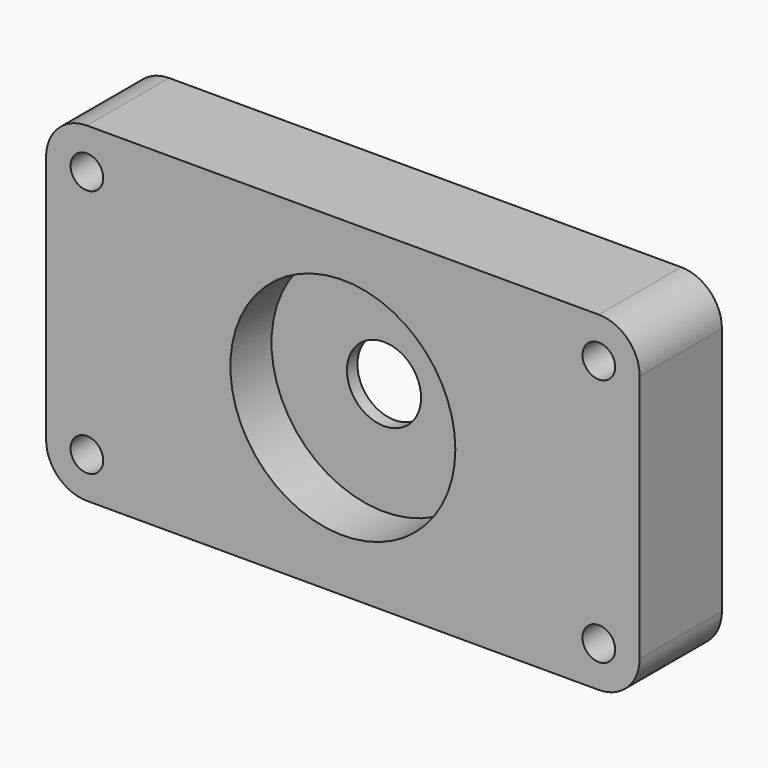
from build123d import *

# Parameters (mm, degrees)
F0_R     = 17.4971354571
F0_R_2   = 11.8450866669
F0_R_3   = 5.7656301988
F1_DEPTH = 2.032
F0_R_4   = 2.5396522034
F2_DEPTH = 8
F3_DEPTH = 8


# Not quite as in the source:
# - a feature names something its author has since deleted; it is built from what else it names


with BuildPart() as f1:
    # F0 (on Front) → F1 (new body)
    with BuildSketch(Plane.XZ):
        with Locations((3.1854841864, -0.0279111721)):
            Circle(F0_R)
        with Locations((3.1854841864, -0.0279111721)):
            Circle(F0_R_2, mode=Mode.SUBTRACT)
        with Locations((3.1854841864, -0.0279111721)):
            Circle(F0_R_2)
        with Locations((3.1854841864, -0.0279111721)):
            Circle(F0_R_3, mode=Mode.SUBTRACT)
    extrude(amount=-F1_DEPTH)

    # F0 (on Front) → F2 (join)
    with BuildSketch(Plane.XZ):
        with BuildLine():
            ThreePointArc((-42.9830769071, -19.3787951119), (-41.1232049677, -23.8689231724), (-36.6330769071, -25.7287951119))
            Line((-36.6330769071, -25.7287951119), (43.0040508678, -25.7287951119))
            ThreePointArc((43.0040508678, -25.7287951119), (47.4941789284, -23.8689231724), (49.3540508678, -19.3787951119))
            Line((49.3540508678, -19.3787951119), (49.3540508678, 19.3229727678))
            ThreePointArc((49.3540508678, 19.3229727678), (47.4941772917, 23.8131047796), (43.0040452799, 25.6729783557))
            Line((43.0040452799, 25.6729783557), (-36.6330769071, 25.6729783557))
            ThreePointArc((-36.6330769071, 25.6729783557), (-41.1232049677, 23.8131064163), (-42.9830769071, 19.3229783557))
            Line((-42.9830769071, 19.3229783557), (-42.9830769071, -19.3787951119))
        make_face()
        with Locations((-36.6330769071, -19.3787951119)):
            Circle(F0_R_4, mode=Mode.SUBTRACT)
        with Locations((3.1854841864, -0.0279111721)):
            Circle(F0_R, mode=Mode.SUBTRACT)
        with Locations((43.0040452799, -19.3787951119)):
            Circle(F0_R_4, mode=Mode.SUBTRACT)
        with Locations((-36.6330769071, 19.3229727678)):
            Circle(F0_R_4, mode=Mode.SUBTRACT)
        with Locations((43.0040452799, 19.3229727678)):
            Circle(F0_R_4, mode=Mode.SUBTRACT)
    extrude(amount=-F2_DEPTH)

    # F0 (on Front) → F3 (join)
    with BuildSketch(Plane.XZ):
        with BuildLine():
            ThreePointArc((-42.9830769071, -19.3787951119), (-41.1232049677, -23.8689231724), (-36.6330769071, -25.7287951119))
            Line((-36.6330769071, -25.7287951119), (43.0040508678, -25.7287951119))
            ThreePointArc((43.0040508678, -25.7287951119), (47.4941789284, -23.8689231724), (49.3540508678, -19.3787951119))
            Line((49.3540508678, -19.3787951119), (49.3540508678, 19.3229727678))
            ThreePointArc((49.3540508678, 19.3229727678), (47.4941772917, 23.8131047796), (43.0040452799, 25.6729783557))
            Line((43.0040452799, 25.6729783557), (-36.6330769071, 25.6729783557))
            ThreePointArc((-36.6330769071, 25.6729783557), (-41.1232049677, 23.8131064163), (-42.9830769071, 19.3229783557))
            Line((-42.9830769071, 19.3229783557), (-42.9830769071, -19.3787951119))
        make_face()
        with Locations((-36.6330769071, -19.3787951119)):
            Circle(F0_R_4, mode=Mode.SUBTRACT)
        with Locations((3.1854841864, -0.0279111721)):
            Circle(F0_R, mode=Mode.SUBTRACT)
        with Locations((43.0040452799, -19.3787951119)):
            Circle(F0_R_4, mode=Mode.SUBTRACT)
        with Locations((-36.6330769071, 19.3229727678)):
            Circle(F0_R_4, mode=Mode.SUBTRACT)
        with Locations((43.0040452799, 19.3229727678)):
            Circle(F0_R_4, mode=Mode.SUBTRACT)
    extrude(amount=F3_DEPTH)


solid = f1.part
